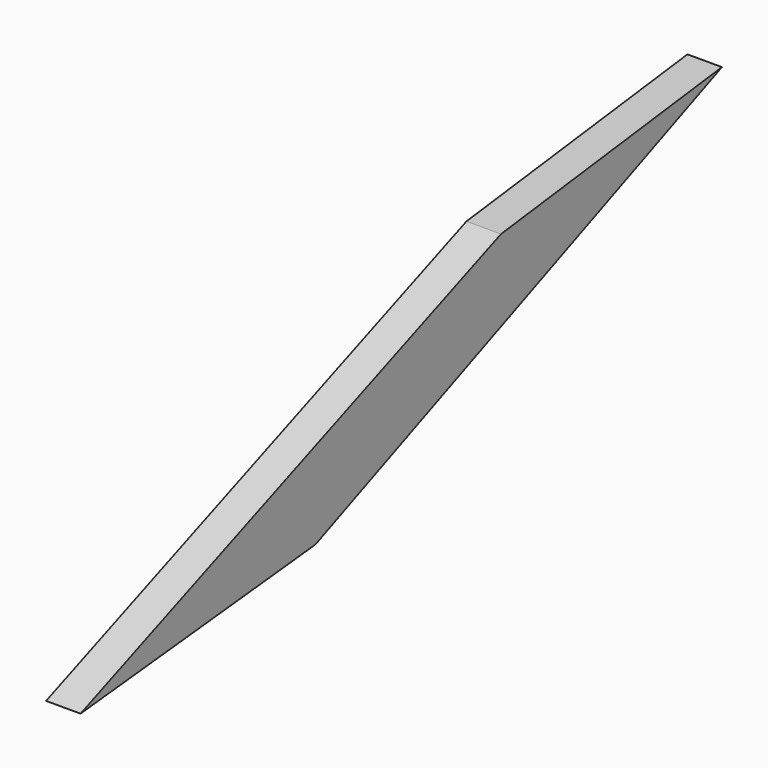
from build123d import *

# Parameters (mm, degrees)
F1_DEPTH = 25


# Not quite as in the source:
# - a feature of the source that left no trace in its solid (it failed there, or was rolled back) is left out


with BuildPart() as f1:
    # F0 (on Right) → F1 (new body)
    with BuildSketch(Plane.YZ):
        Polygon((-368.2365715504, -154.8998206854), (0, 0), (-200.1617848873, -25.162473321), (-580.9631347656, -176.3214021921), align=None)
    extrude(amount=F1_DEPTH)


solid = f1.part
